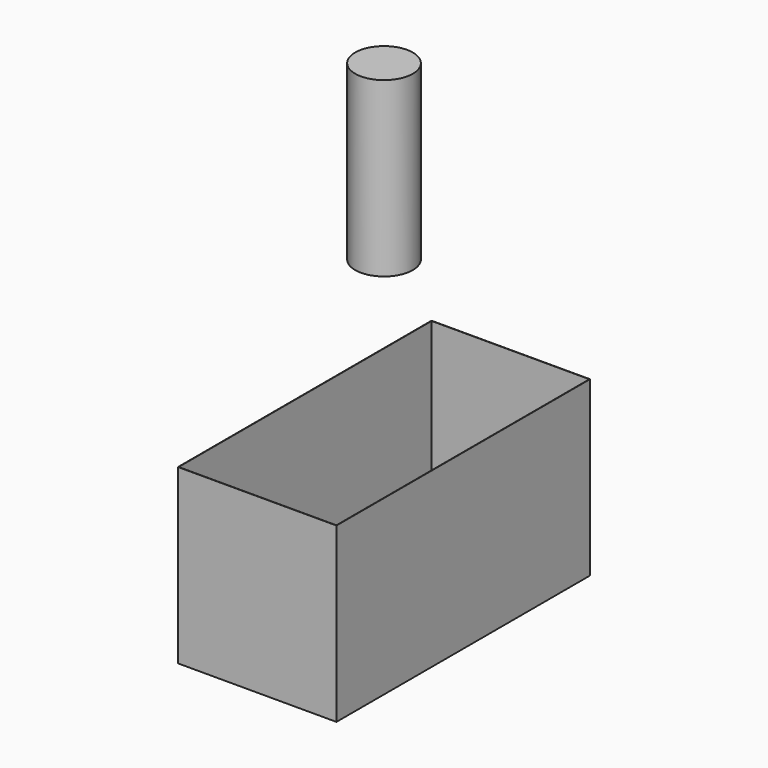
from build123d import *

# Parameters (mm, degrees)
F0_W      = 279.4
F0_H      = 558.8
F0_W_2    = 278.1808
F0_H_2    = 557.5808
F1_DEPTH  = 304.8
F10_R     = 50.8
F11_DEPTH = 304.8


# Not quite as in the source:
# - the program builds the solid bodies; features that only make, move or delete a surface that nothing else refers to are left out


with BuildPart() as f1:
    # F0 (on Top) → F1 (new body)
    with BuildSketch(Plane.XY):
        with Locations((139.7, 279.4)):
            Rectangle(F0_W, F0_H)
        with Locations((139.7, 279.4)):
            Rectangle(F0_W_2, F0_H_2, mode=Mode.SUBTRACT)
    extrude(amount=F1_DEPTH)


with BuildPart() as f11:
    # F10 (on offset) → F11 (new body)
    with BuildSketch(Plane.XY.offset(558.8)):
        with Locations((139.7, 279.4)):
            Circle(F10_R)
    extrude(amount=F11_DEPTH)


solid = Compound([f1.part, f11.part])
